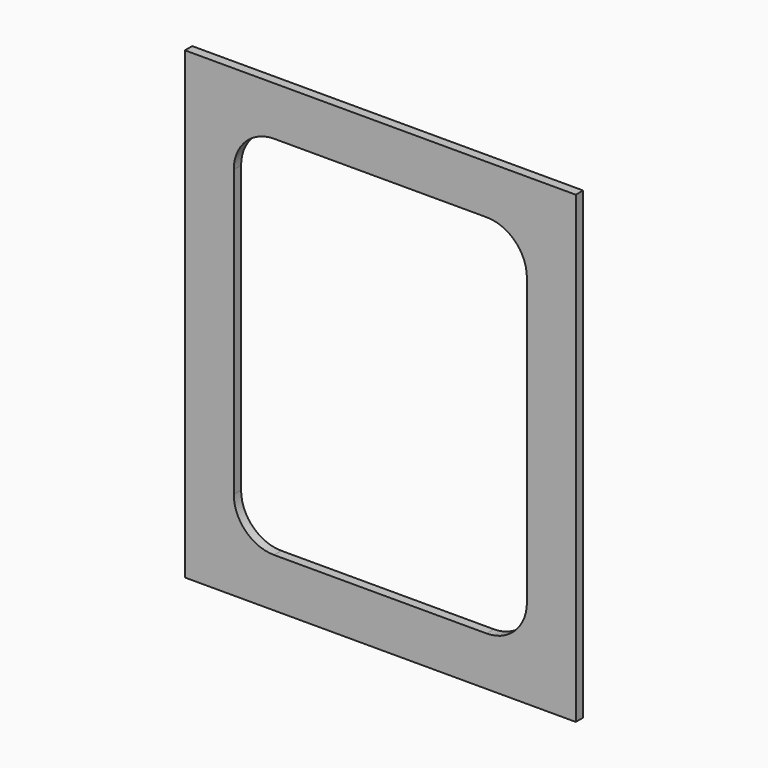
from build123d import *

# Parameters (mm, degrees)
F0_W     = 406.4
F0_H     = 482.6
F1_DEPTH = 9.525


# Not quite as in the source:
# - a length typed as a fraction of an inch, garbled in the dataset ("3 / 203.2 mm" for 3/8 in), is restored


with BuildPart() as f1:
    # F0 (on Front) → F1 (new body)
    with BuildSketch(Plane.XZ):
        with Locations((-135.2954388559, 273.8481773734)):
            Rectangle(F0_W, F0_H)
        with BuildLine():
            ThreePointArc((17.1045611441, 125.2581773734), (4.8294063436, 95.6233321739), (-24.8054388559, 83.3481773734))
            Line((-24.8054388559, 83.3481773734), (-245.7854388559, 83.3481773734))
            ThreePointArc((-245.7854388559, 83.3481773734), (-275.4202840554, 95.6233321739), (-287.6954388559, 125.2581773734))
            Line((-287.6954388559, 125.2581773734), (-287.6954388559, 422.4381773734))
            ThreePointArc((-287.6954388559, 422.4381773734), (-275.4202840554, 452.0730225729), (-245.7854388559, 464.3481773734))
            Line((-245.7854388559, 464.3481773734), (-24.8054388559, 464.3481773734))
            ThreePointArc((-24.8054388559, 464.3481773734), (4.8294063436, 452.0730225729), (17.1045611441, 422.4381773734))
            Line((17.1045611441, 422.4381773734), (17.1045611441, 125.2581773734))
        make_face(mode=Mode.SUBTRACT)
    extrude(amount=F1_DEPTH)


solid = f1.part
